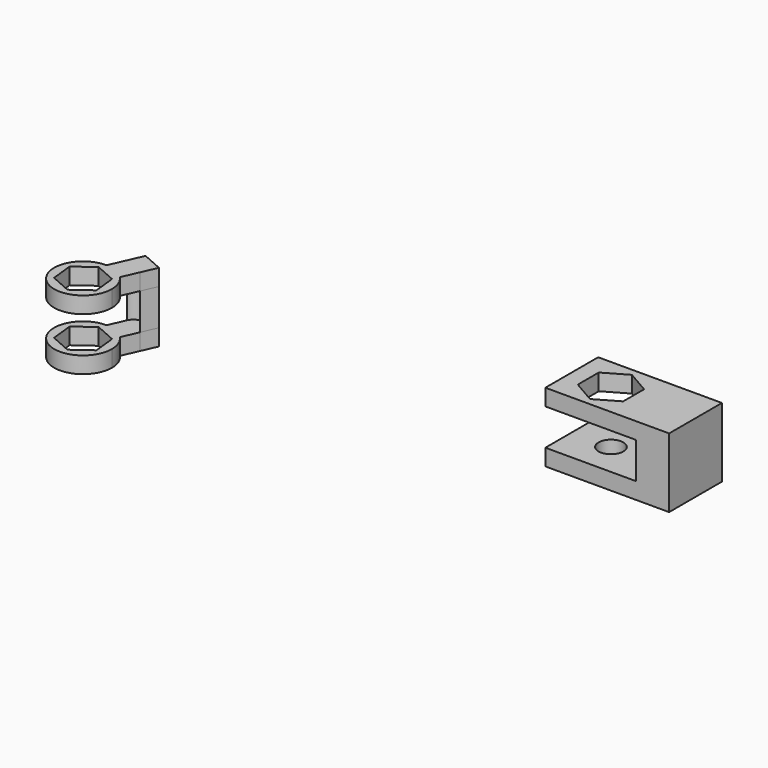
from build123d import *

# Parameters (mm, degrees)
F1_DEPTH  = 8.4
F3_DEPTH  = 25
F4_W      = 9.4060590708
F4_H      = 4.4
F5_DEPTH  = 25
F7_DEPTH  = 4.4
F8_W      = 15
F8_H      = 8
F9_DEPTH  = 10
F10_W     = 11
F10_H     = 4.4
F11_DEPTH = 25
F12_W     = 15
F12_H     = 1.6
F13_DEPTH = 25
F14_DEPTH = 10
F15_R     = 1.5
F16_DEPTH = 25


# Not quite as in the source:
# - a feature names something its author has since deleted; it is built from what else it names


with BuildPart() as f1:
    # F0 (on Top) → F1 (new body)
    with BuildSketch(Plane.XY):
        with BuildLine():
            Line((-17.517138558, 6.0693021001), (-17.8563866138, 5.3041045041))
            Line((-17.8563866138, 5.3041045041), (-17.5646357736, 2.5696243986))
            Line((-17.5646357736, 2.5696243986), (-19.786889591, 0.9497207067))
            Line((-19.786889591, 0.9497207067), (-22.3008942486, 2.0642971202))
            Line((-22.3008942486, 2.0642971202), (-22.5926450887, 4.7987772257))
            Line((-22.5926450887, 4.7987772257), (-20.3703912714, 6.4186809176))
            Line((-20.3703912714, 6.4186809176), (-20.0311432156, 7.1838785137))
            ThreePointArc((-20.0311432156, 7.1838785137), (-22.570250378, 1.2261772417), (-16.5786404312, 3.6842008121))
            ThreePointArc((-16.5786404312, 3.6842008121), (-16.8217050192, 4.9657513269), (-17.517138558, 6.0693021001))
        make_face()
        with BuildLine():
            Line((-20.3703912714, 6.4186809176), (-17.8563866138, 5.3041045041))
            Line((-17.8563866138, 5.3041045041), (-17.517138558, 6.0693021001))
            ThreePointArc((-17.517138558, 6.0693021001), (-18.6600886321, 6.8838431036), (-20.0311432156, 7.1838785137))
            Line((-20.0311432156, 7.1838785137), (-20.3703912714, 6.4186809176))
        make_face()
        with BuildLine():
            ThreePointArc((-20.0311432156, 7.1838785137), (-18.6600886321, 6.8838431036), (-17.517138558, 6.0693021001))
            Line((-17.517138558, 6.0693021001), (-16.6404850717, 8.0466550396))
            ThreePointArc((-16.6404850717, 8.0466550396), (-17.3401991937, 9.8609455752), (-19.1544897293, 9.1612314532))
            Line((-19.1544897293, 9.1612314532), (-20.0311432156, 7.1838785137))
        make_face()
        with BuildLine():
            ThreePointArc((-19.1544897293, 9.1612314532), (-17.3401991937, 9.8609455752), (-16.6404850717, 8.0466550396))
            Line((-16.6404850717, 8.0466550396), (-15.8298840437, 9.8750220633))
            Line((-15.8298840437, 9.8750220633), (-18.3438887013, 10.9895984768))
            Line((-18.3438887013, 10.9895984768), (-19.1544897293, 9.1612314532))
        make_face()
    extrude(amount=F1_DEPTH)

    # F2 (on face) → F3 (cut)
    with BuildSketch(Plane(origin=(-16.8884163977, 7.4874286817, 0), x_dir=(0.405300514, 0.9141835118, 0), z_dir=(0.9141835118, -0.405300514, 0))):
        Polygon((-1.5512493534, 2), (2.6117222096, 2), (2.6117222096, 6.4), (-1.5512493534, 6.4), (-9.2430952936, 6.4), (-9.2430952936, 2), align=None)
    extrude(amount=-F3_DEPTH, mode=Mode.SUBTRACT)

    # F4 (on face) → F5 (cut)
    with BuildSketch(Plane(origin=(-16.8884163977, 7.4874286817, 0), x_dir=(-0.405300514, -0.9141835118, 0), z_dir=(-0.9141835118, 0.405300514, 0))):
        with Locations((3.2854164128, 4.2)):
            Rectangle(F4_W, F4_H)
    extrude(amount=-F5_DEPTH, mode=Mode.SUBTRACT)


with BuildPart() as f7:
    # F6 (on face) → F7 (new body)
    with BuildSketch(Plane.XY.offset(2)):
        with BuildLine():
            Line((-18.3438887013, 10.9895984768), (-19.1544897293, 9.1612314532))
            ThreePointArc((-19.1544897293, 9.1612314532), (-17.3401991937, 9.8609455752), (-16.6404850717, 8.0466550396))
            Line((-16.6404850717, 8.0466550396), (-15.8298840437, 9.8750220633))
            Line((-15.8298840437, 9.8750220633), (-18.3438887013, 10.9895984768))
        make_face()
    extrude(amount=F7_DEPTH)


with BuildPart() as f9:
    # F8 (on Top) → F9 (new body)
    with BuildSketch(Plane.XY):
        with Locations((37.5055125356, 15.1265042797)):
            Rectangle(F8_W, F8_H)
        Polygon((32.0055125356, 13.5387910394), (32.0055125356, 16.7142175199), (34.7555125356, 18.3019307602), (37.5055125356, 16.7142175199), (37.5055125356, 13.5387910394), (34.7555125356, 11.9510777991), align=None, mode=Mode.SUBTRACT)
    extrude(amount=F9_DEPTH)

    # F10 (on face) → F11 (cut)
    with BuildSketch(Plane.XZ.offset(-11.1265042797)):
        with Locations((35.5055125356, 5.8)):
            Rectangle(F10_W, F10_H)
    extrude(amount=-F11_DEPTH, mode=Mode.SUBTRACT)

    # F12 (on face) → F13 (cut)
    with BuildSketch(Plane(origin=(0, 19.1265042797, 0), x_dir=(-1, 0, 0), z_dir=(0, 1, 0))):
        with Locations((-37.5055125356, 0.8)):
            Rectangle(F12_W, F12_H)
    extrude(amount=-F13_DEPTH, mode=Mode.SUBTRACT)

    # F14 (add): a face of the model
    f14_faces = [f9.faces().sort_by_distance(p)[0] for p in [
        (30.0055125356, 15.1265042797, 2.6),
    ]]
    extrude(f14_faces, amount=-F14_DEPTH)

    # F15 (on face) → F16 (cut)
    with BuildSketch(Plane(origin=(0, 0, 1.6), x_dir=(1, 0, 0), z_dir=(0, 0, -1))):
        with Locations((34.7555125356, -15.1265042797)):
            Circle(F15_R)
    extrude(amount=-F16_DEPTH, mode=Mode.SUBTRACT)


solid = Compound([f1.part, f7.part, f9.part])
